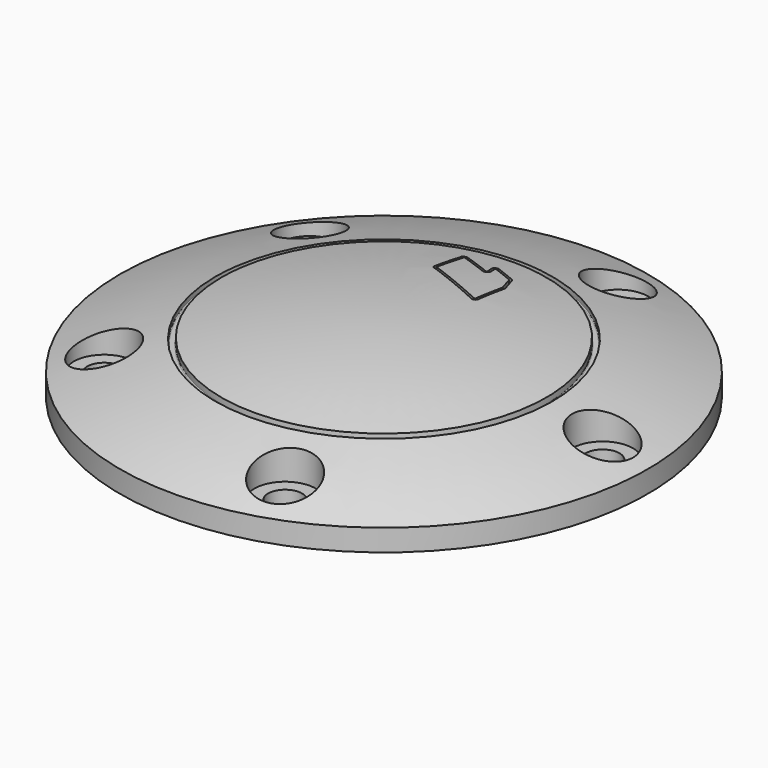
from build123d import *

# Parameters (mm, degrees)
F2_R            = 2.4765
F3_DEPTH        = 10.161
F3_COPIES_COUNT = 5
F5_R            = 4.445
F6_DEPTH        = 25.4
F6_COPIES_COUNT = 5
F13_W           = 0.381
F13_H           = 20.32


# Not quite as in the source:
# - a pattern or mirror of a feature is missing from the dataset's text; its kind, count and spacing are read off the source's solid


with BuildPart() as f1:
    # F0 (on Front) → F1 (revolve)
    with BuildSketch(Plane.XZ):
        with BuildLine():
            Line((0, 99.3301636364), (0, 109.4901636364))
            ThreePointArc((0, 109.4901636364), (-19.554907223, 107.7297616103), (-38.481, 102.5051636364))
            Line((-38.481, 102.5051636364), (-38.481, 99.3301636364))
            Line((-38.481, 99.3301636364), (0, 99.3301636364))
        make_face()
    revolve(axis=Axis((0, 0, 54.7450818182), (0, 0, -1)))

    # F2 (on face) → F3 (cut, through all)
    with BuildSketch(Plane(origin=(0, 0, 99.3301636364), x_dir=(1, 0, 0), z_dir=(0, 0, -1))):
        with Locations((31.877, 0)):
            Circle(F2_R)
    f3 = extrude(amount=-F3_DEPTH, mode=Mode.SUBTRACT)

    # F3_copies: F3 ×5 about axis
    f3_copies_axis = Axis((0, 0, 0), (0, 0, 1))
    for i in range(1, F3_COPIES_COUNT):
        add(f3.rotate(f3_copies_axis, i * 360 / F3_COPIES_COUNT), mode=Mode.SUBTRACT)

    # F5 (on offset) → F6 (cut)
    with BuildSketch(Plane.XY.offset(101.6)):
        with Locations((31.877, 0)):
            Circle(F5_R)
    f6 = extrude(amount=F6_DEPTH, mode=Mode.SUBTRACT)

    # F6_copies: F6 ×5 about axis
    f6_copies_axis = Axis((0, 0, 0), (0, 0, 1))
    for i in range(1, F6_COPIES_COUNT):
        add(f6.rotate(f6_copies_axis, i * 360 / F6_COPIES_COUNT), mode=Mode.SUBTRACT)

    # F8 (on Right) → F9 (revolve, cut)
    with BuildSketch(Plane.YZ):
        with BuildLine():
            Line((24.5872, 116.0843521357), (23.6982, 116.0843521357))
            Line((23.6982, 116.0843521357), (23.6982, 106.0611636364))
            ThreePointArc((23.6982, 106.0611636364), (23.7353974388, 105.9713610752), (23.8252, 105.9341636364))
            Line((23.8252, 105.9341636364), (24.4602, 105.9341636364))
            ThreePointArc((24.4602, 105.9341636364), (24.5500025612, 105.9713610752), (24.5872, 106.0611636364))
            Line((24.5872, 106.0611636364), (24.5872, 116.0843521357))
        make_face()
    revolve(axis=Axis((0, 0, 96.7393070459), (0, 0, 1)), mode=Mode.SUBTRACT)

    # F14: sweep along a path in F11
    with BuildLine(Plane.XY.offset(127)) as f14_path:
        ThreePointArc((-4.445, 15.2089718991), (-4.4251107136, 15.1407348489), (-4.3716725192, 15.0938708102))
        Line((-4.3716725192, 15.0938708102), (4.2643274808, 11.0668378744))
        ThreePointArc((4.2643274808, 11.0668378744), (4.3862370503, 11.0748282497), (4.445, 11.1819389633))
        Line((4.445, 11.1819389633), (4.445, 15.9871306382))
        ThreePointArc((4.445, 15.9871306382), (4.4377405074, 16.0611511295), (4.4162386712, 16.1323508796))
        Line((4.4162386712, 16.1323508796), (3.4625941664, 18.4454614342))
        ThreePointArc((3.4625941664, 18.4454614342), (3.3857938611, 18.5634800702), (3.271373053, 18.6455444596))
        Line((3.271373053, 18.6455444596), (0.4623161154, 19.9554292218))
        ThreePointArc((0.4623161154, 19.9554292218), (0.3285349542, 19.9388756111), (0.2850066214, 19.8112954192))
        Line((0.2850066214, 19.8112954192), (0.52275878, 18.7988183233))
        ThreePointArc((0.52275878, 18.7988183233), (0.3486454489, 18.2884975555), (-0.1864791961, 18.2222831127))
        Line((-0.1864791961, 18.2222831127), (-4.2643274808, 20.1238149967))
        ThreePointArc((-4.2643274808, 20.1238149967), (-4.3862370503, 20.1158246213), (-4.445, 20.0087139077))
        Line((-4.445, 20.0087139077), (-4.445, 15.2089718991))
    # F13 (on plane+point) → F14 (sweep, cut)
    with BuildSketch(Plane.YZ.offset(-4.3716725192)):
        with Locations((14.9033708102, 116.84)):
            Rectangle(F13_W, F13_H)
    sweep(path=f14_path.line, mode=Mode.SUBTRACT)


solid = f1.part
